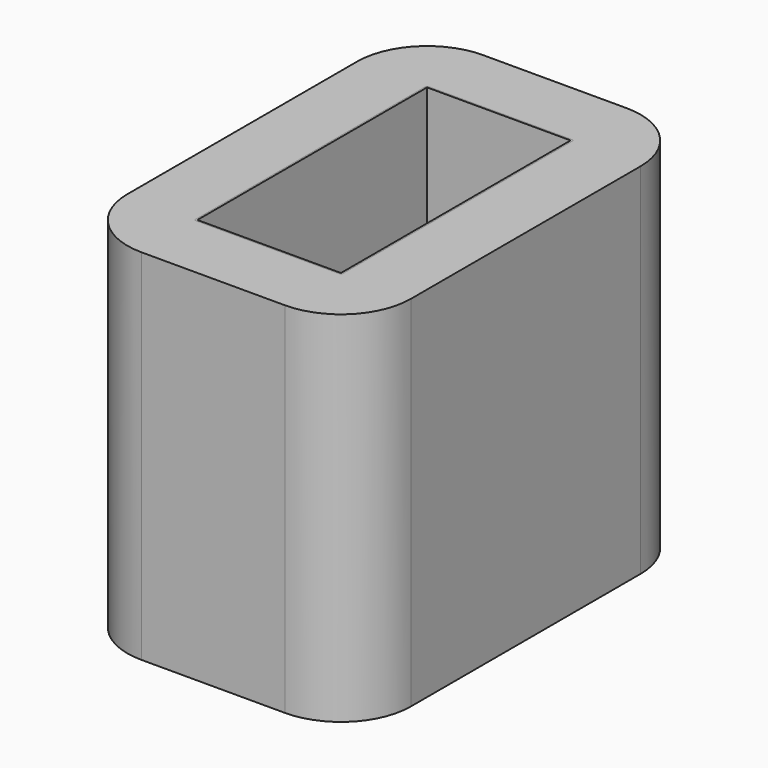
from build123d import *

# Parameters (mm, degrees)
F4_W      = 120.396
F4_H      = 181.356
F5_DEPTH  = 152.4
F6_R      = 29.718
F7_W      = 62.484
F7_H      = 123.444
F8_DEPTH  = 152.4
F9_W      = 62.484
F9_H      = 123.444
F10_DEPTH = 152.4
F11_W     = 60.96
F11_H     = 121.92
F12_DEPTH = 152.4
F13_R     = 0.762
F14_R     = 0.762


with BuildPart() as f5:
    # F4 (on Top) → F5 (new body)
    with BuildSketch(Plane.XY):
        Rectangle(F4_W, F4_H)
    extrude(amount=-F5_DEPTH)

    # F6
    f6_edges = [f5.edges().sort_by_distance(p)[0] for p in [
        (-60.198, 90.678, -76.2),
        (60.198, 90.678, -76.2),
        (60.198, -90.678, -76.2),
        (-60.198, -90.678, -76.2),
    ]]
    fillet(f6_edges, radius=F6_R)

    # F7 (on face) → F8 (cut)
    with BuildSketch(Plane.XY):
        Rectangle(F7_W, F7_H)
    extrude(amount=-F8_DEPTH, mode=Mode.SUBTRACT)

    # F14
    f14_edges = [f5.edges().sort_by_distance(p)[0] for p in [
        (-31.242, 61.722, -76.2),
        (-31.242, -61.722, -76.2),
        (31.242, -61.722, -76.2),
        (31.242, 61.722, -76.2),
    ]]
    fillet(f14_edges, radius=F14_R)


with BuildPart() as f10:
    # F9 (on face) → F10 (new body)
    with BuildSketch(Plane.XY):
        Rectangle(F9_W, F9_H)
    extrude(amount=-F10_DEPTH)

    # F11 (on face) → F12 (cut)
    with BuildSketch(Plane.XY):
        Rectangle(F11_W, F11_H)
    extrude(amount=-F12_DEPTH, mode=Mode.SUBTRACT)

    # F13
    f13_edges = [f10.edges().sort_by_distance(p)[0] for p in [
        (-31.242, 61.722, -76.2),
        (31.242, 61.722, -76.2),
        (31.242, -61.722, -76.2),
        (-31.242, -61.722, -76.2),
    ]]
    fillet(f13_edges, radius=F13_R)


solid = Compound([f5.part, f10.part])
